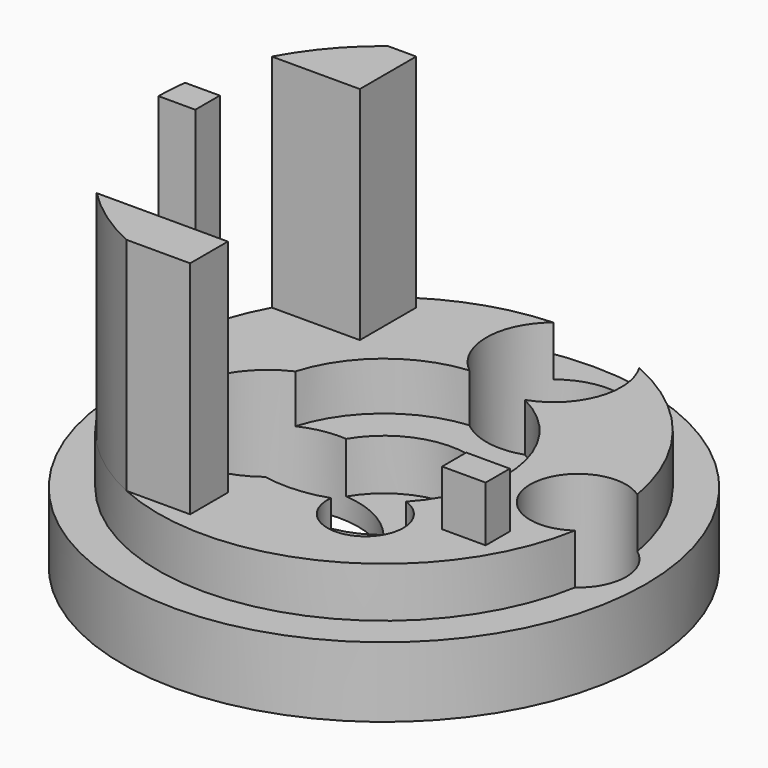
from build123d import *

# Parameters (mm, degrees)
F2_R     = 21.6962130455
F2_R_2   = 17.1617704493
F2_R_3   = 40.953196501
F2_R_4   = 30.4988959279
F3_DEPTH = 1000
F5_DEPTH = 100
F6_W     = 19.7006091475
F6_H     = 13.662148267
F7_DEPTH = 25


# Not quite as in the source:
# - after a boolean that leaves OpenCascade's solid faulty, fix() repairs it


with BuildPart() as f1:
    # F0 (on Front) → F1 (revolve)
    with BuildSketch(Plane.XZ):
        Polygon((0, 9.6338680014), (0, 0), (118.4682399035, 0), (118.4682399035, 31.7357704043), (102.0300611854, 31.7357704043), (102.0300611854, 54.4380694628), (54.9828708172, 54.4380694628), (54.9828708172, 32.5937792659), (37.9778593779, 32.5937792659), (37.9778593779, 9.6338680014), align=None)
    revolve(axis=Axis((0, 0, 4.8169340007), (0, 0, -1)))

    # F2 (on face) → F3 (cut)
    with BuildSketch(Plane(origin=(0, 0, 0), x_dir=(1, 0, 0), z_dir=(0, 0, -1))):
        with Locations((87.8278240561, 0)):
            Circle(F2_R)
        with Locations((34.7668491304, 54.0037713945)):
            Circle(F2_R_2)
        with Locations((-35.4811474681, 21.4303005487)):
            Circle(F2_R_3)
        with Locations((14.2781008035, -78.1974196434)):
            Circle(F2_R_4)
    extrude(amount=-F3_DEPTH, mode=Mode.SUBTRACT)

    # F4 (on face) → F5 (join)
    with BuildSketch(Plane.XY.offset(54.4380694628)):
        with BuildLine():
            Line((-49.8583316803, 48.6504090547), (-49.8583316803, 80.5302113295))
            Line((-49.8583316803, 80.5302113295), (-62.6499676674, 80.5302113295))
            ThreePointArc((-62.6499676674, 80.5302113295), (-77.8171679529, 65.9895579412), (-89.684285604, 48.6504090547))
            Line((-89.684285604, 48.6504090547), (-49.8583316803, 48.6504090547))
        make_face()
        with BuildLine():
            Line((-85.3846818209, 13.8626152044), (-101.0839318843, 13.8626152044))
            ThreePointArc((-101.0839318843, 13.8626152044), (-101.7932540508, 6.9474322767), (-102.0300611854, 0))
            Line((-102.0300611854, 0), (-85.3846818209, 0))
            Line((-85.3846818209, 0), (-85.3846818209, 13.8626152044))
        make_face()
        with BuildLine():
            Line((-13.3902756497, -71.5824663639), (-72.7054598689, -71.5824663639))
            ThreePointArc((-72.7054598689, -71.5824663639), (-58.4249180154, -83.6460539439), (-42.1830749936, -92.9016768932))
            Line((-42.1830749936, -92.9016768932), (-13.3902756497, -92.9016768932))
            Line((-13.3902756497, -92.9016768932), (-13.3902756497, -71.5824663639))
        make_face()
    extrude(amount=F5_DEPTH)

    add(f1.part.fix(), mode=Mode.REPLACE)

    # F6 (on face) → F7 (join)
    with BuildSketch(Plane.XY.offset(54.4380694628)):
        with Locations((73.1044746935, -39.3697526306)):
            Rectangle(F6_W, F6_H)
    extrude(amount=F7_DEPTH)


solid = f1.part
